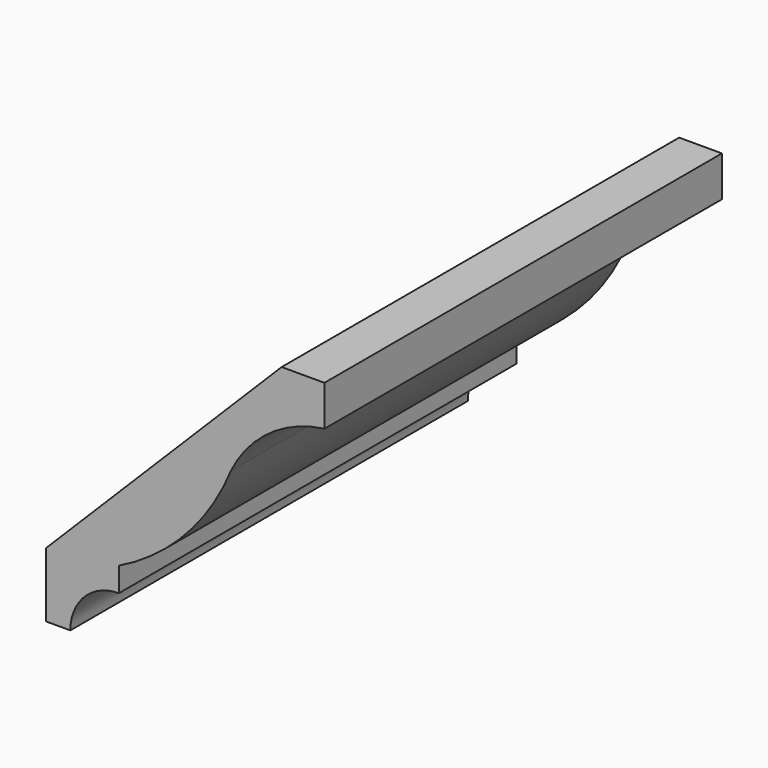
from build123d import *

# Parameters (mm, degrees)
F1_DEPTH = 152.4


# Not quite as in the source:
# - ends of sketch curves that miss each other by under 0.0002 mm in the source are joined


with BuildPart() as f1:
    # F0 (on Front) → F1 (new body)
    with BuildSketch(Plane.XZ):
        with BuildLine():
            Line((42.688764, 33.7040728), (42.688764, 46.1017112))
            Line((42.688764, 46.1017112), (29.5671748, 46.1017112))
            Line((29.5671748, 46.1017112), (-42.688764, -26.265505))
            Line((-42.688764, -26.265505), (-42.688764, -46.1017112))
            Line((-42.688764, -46.1017112), (-35.2501708, -46.1017112))
            ThreePointArc((-35.2501708, -46.1017112), (-30.8927586674, -35.5819877326), (-20.3730352, -31.2245756))
            Line((-20.3730352, -31.2245756), (-20.3730352, -23.7859824))
            ThreePointArc((-20.3730352, -23.7859824), (0.2093797229, -8.5380689207), (14.0097452821, 13.0416577293))
            ThreePointArc((14.0097452821, 13.0416577293), (25.7531505711, 26.9762086577), (42.688764, 33.7040728))
        make_face()
    extrude(amount=F1_DEPTH)


solid = f1.part
